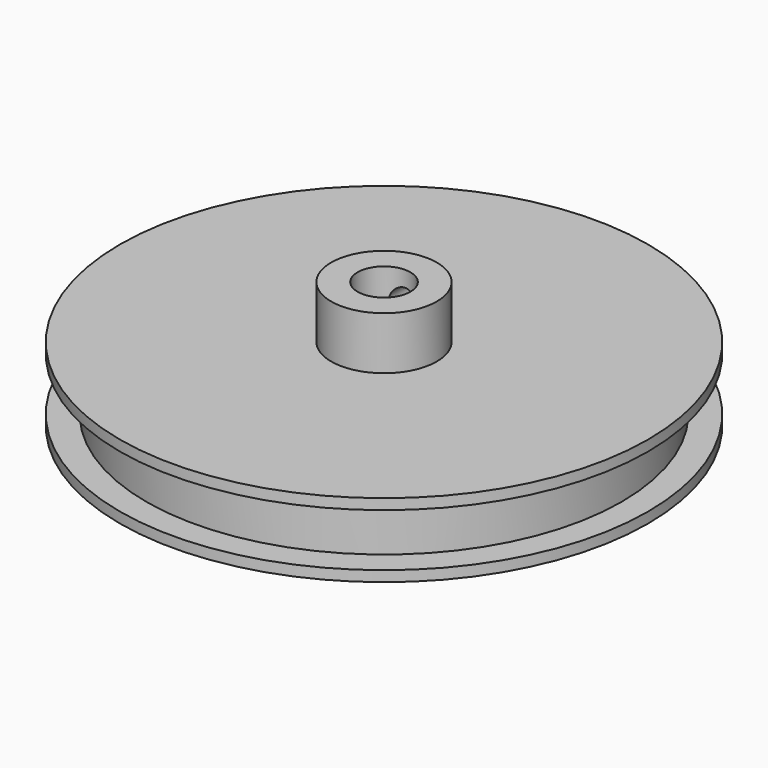
from build123d import *

# Parameters (mm, degrees)
F0_R      = 50
F1_DEPTH  = 2
F2_R      = 45
F3_DEPTH  = 10
F4_R      = 50
F4_R_2    = 45
F5_DEPTH  = 2
F6_R      = 10
F7_DEPTH  = 10
F8_R      = 10
F9_DEPTH  = 10
F10_R     = 5
F11_DEPTH = 34.001
F14_R     = 2.5
F15_DEPTH = 6.6698730813


with BuildPart() as f1:
    # F0 (on Top) → F1 (new body)
    with BuildSketch(Plane.XY):
        Circle(F0_R)
    extrude(amount=F1_DEPTH)

    # F2 (on face) → F3 (join)
    with BuildSketch(Plane.XY.offset(2)):
        Circle(F2_R)
    extrude(amount=F3_DEPTH)

    # F4 (on face) → F5 (join)
    with BuildSketch(Plane.XY.offset(12)):
        Circle(F4_R)
        Circle(F4_R_2, mode=Mode.SUBTRACT)
        Circle(F4_R_2)
    extrude(amount=F5_DEPTH)

    # F6 (on face) → F7 (join)
    with BuildSketch(Plane.XY.offset(14)):
        Circle(F6_R)
    extrude(amount=F7_DEPTH)

    # F8 (on face) → F9 (join)
    with BuildSketch(Plane(origin=(0, 0, 0), x_dir=(1, 0, 0), z_dir=(0, 0, -1))):
        Circle(F8_R)
    extrude(amount=F9_DEPTH)

    # F10 (on face) → F11 (cut, through all)
    with BuildSketch(Plane.XY.offset(24)):
        Circle(F10_R)
    extrude(amount=-F11_DEPTH, mode=Mode.SUBTRACT)

    # F14 (on face) → F15 (cut, up to face)
    with BuildSketch(Plane(origin=(0, 10, 0), x_dir=(-1, 0, 0), z_dir=(0, 1, 0))):
        with Locations((0, 18.5063882234)):
            Circle(F14_R)
        with Locations((0, -5.5)):
            Circle(F14_R)
    extrude(amount=-F15_DEPTH, mode=Mode.SUBTRACT)


solid = f1.part
